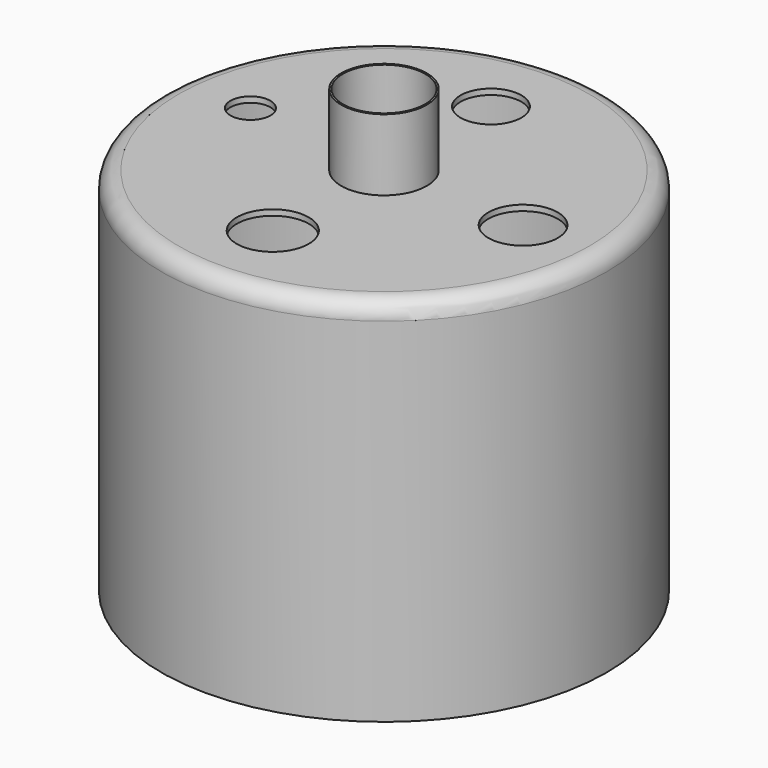
from build123d import *

# Parameters (mm, degrees)
F0_R           = 27.051
F2_R           = 33.02
F4_DEPTH       = 112.522
F8_DEPTH       = 25.4
F6_R           = 31.8662185307
F10_R          = 27.1012036097
F12_DEPTH      = 111.67649
F13_R          = 6.35
F13_R_2        = 6.096
F14_DEPTH      = 25.4
F15_DEPTH      = 25.4
F16_W          = 95.3798592091
F16_H          = 79.9988703802
F17_DEPTH      = 50.8
F17_DEPTH_BACK = 50.8
F18_R          = 4.5084907347
F18_R_2        = 5.1462074836
F18_R_3        = 5.3392585876
F18_R_4        = 2.9616888365
F19_DEPTH      = 25.4
F20_R          = 2.54
F21_W          = 29.3621988967
F21_H          = 16.516238451
F22_DEPTH      = 25.4
F22_DEPTH_BACK = 25.4


with BuildPart() as f3:
    # F0 (on Top) → F3 section 0
    with BuildSketch(Plane.XY):
        Circle(F0_R)
    # F2 (on offset) → F3 section 1
    with BuildSketch(Plane.XY.offset(10.16)):
        Circle(F2_R)
    loft()

    # F4 (add): a face of the model
    f4_faces = [f3.faces().sort_by_distance(p)[0] for p in [
        (0, 0, 10.16),
    ]]
    extrude(f4_faces, amount=F4_DEPTH)

    # F7 (on face) → F8 (cut)
    with BuildSketch(Plane(origin=(0, 0, 0), x_dir=(1, 0, 0), z_dir=(0, 0, -1))):
        with BuildLine():
            Line((-9.0020672118, 14.5257171748), (8.9738084456, 14.5257171748))
            ThreePointArc((8.9738084456, 14.5257171748), (-0.0141293831, 22.7222466067), (-9.0020672118, 14.5257171748))
        make_face()
    extrude(amount=-F8_DEPTH, mode=Mode.SUBTRACT)

    # F6 (on offset) → F11 section 0
    with BuildSketch(Plane.XY.offset(10.16)):
        Circle(F6_R)
    # F10 (on offset) → F11 section 1
    with BuildSketch(Plane(origin=(0, 0, 1.016), x_dir=(1, 0, 0), z_dir=(0, 0, -1))):
        Circle(F10_R)
    loft(mode=Mode.SUBTRACT)

    # F6 (on offset) → F12 (cut)
    with BuildSketch(Plane.XY.offset(10.16)):
        Circle(F6_R)
    extrude(amount=F12_DEPTH, mode=Mode.SUBTRACT)

    # F13 (on face) → F14 (join)
    with BuildSketch(Plane.XY.offset(122.682)):
        Circle(F13_R)
        Circle(F13_R_2, mode=Mode.SUBTRACT)
    extrude(amount=F14_DEPTH)

    # F15 (cut): a face of the model
    f15_faces = [f3.faces().sort_by_distance(p)[0] for p in [
        (0, 0, 122.682),
    ]]
    extrude(f15_faces, amount=-F15_DEPTH, mode=Mode.SUBTRACT)

    # F16 (on Right) → F17 (cut, two sides)
    with BuildSketch(Plane.YZ) as f17_sk:
        with Locations((3.9506442845, 27.8317159973)):
            Rectangle(F16_W, F16_H)
    extrude(amount=-F17_DEPTH, mode=Mode.SUBTRACT)
    extrude(f17_sk.sketch, amount=F17_DEPTH_BACK, mode=Mode.SUBTRACT)

    # F18 (on face) → F19 (cut)
    with BuildSketch(Plane.XY.offset(122.682)):
        with Locations((-0.2904168505, 20.1840121299)):
            Circle(F18_R)
        with Locations((21.2004743516, -0.7260435959)):
            Circle(F18_R_2)
        with Locations((-0.5808342248, -19.8935940862)):
            Circle(F18_R_3)
        with Locations((-21.7813067138, 2.4685480166)):
            Circle(F18_R_4)
    extrude(amount=-F19_DEPTH, mode=Mode.SUBTRACT)

    # F20
    f20_edges = [f3.edges().sort_by_distance(p)[0] for p in [
        (-33.02, 0, 122.682),
    ]]
    fillet(f20_edges, radius=F20_R)

    # F21 (on Front) → F22 (cut, two sides)
    with BuildSketch(Plane.XZ) as f22_sk:
        with Locations((0.4587839358, 141.5242999792)):
            Rectangle(F21_W, F21_H)
    extrude(amount=-F22_DEPTH, mode=Mode.SUBTRACT)
    extrude(f22_sk.sketch, amount=F22_DEPTH_BACK, mode=Mode.SUBTRACT)


solid = f3.part
